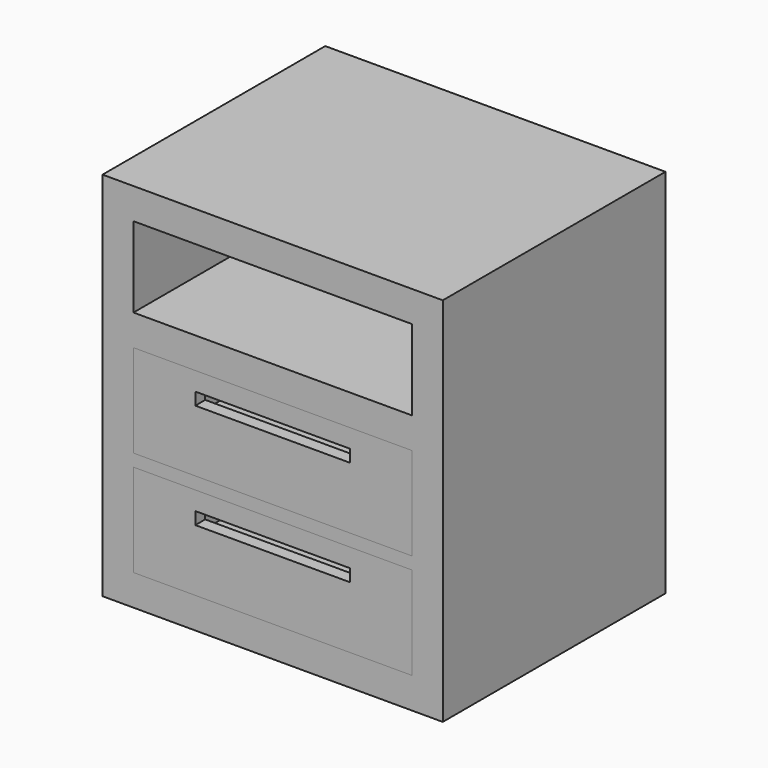
from build123d import *

# Parameters (mm, degrees)
F0_W     = 550
F0_H     = 450
F1_DEPTH = 600
F2_W     = 450
F2_H     = 150
F2_H_2   = 130
F3_DEPTH = 430
F4_DEPTH = 20.001
F5_DEPTH = 430
F6_T     = -20
F6_2_T   = -20
F7_W     = 250
F7_H     = 20
F8_DEPTH = 20


with BuildPart() as f1:
    # F0 (on Top) → F1 (new body)
    with BuildSketch(Plane.XY):
        Rectangle(F0_W, F0_H)
    extrude(amount=F1_DEPTH)

    # F2 (on face) → F3 (cut)
    with BuildSketch(Plane.XZ.offset(225)):
        with Locations((0, 125)):
            Rectangle(F2_W, F2_H)
        with Locations((0, 295)):
            Rectangle(F2_W, F2_H)
        with Locations((0, 485)):
            Rectangle(F2_W, F2_H_2)
    extrude(amount=-F3_DEPTH, mode=Mode.SUBTRACT)

    # F4 (cut, through all): a face of the model
    f4_faces = [f1.faces().sort_by_distance(p)[0] for p in [
        (0, 205, 485),
    ]]
    extrude(f4_faces, amount=-F4_DEPTH, mode=Mode.SUBTRACT)


with BuildPart() as f5:
    # F2 (on face) → F5 (new body, through all)
    with BuildSketch(Plane.XZ.offset(225)):
        with Locations((0, 125)):
            Rectangle(F2_W, F2_H)
    extrude(amount=-F5_DEPTH)

    # F6#2
    f6_2_openings = [f5.faces().sort_by_distance(p)[0] for p in [
        (0, -10, 200),
    ]]
    offset(amount=F6_2_T, openings=f6_2_openings)


with BuildPart() as f5b:
    # F2 (on face) → F5, piece 2 (new body, through all)
    with BuildSketch(Plane.XZ.offset(225)):
        with Locations((0, 295)):
            Rectangle(F2_W, F2_H)
    extrude(amount=-F5_DEPTH)

    # F6
    f6_openings = [f5b.faces().sort_by_distance(p)[0] for p in [
        (0, -10, 370),
    ]]
    offset(amount=F6_T, openings=f6_openings)


with BuildPart() as f8_tool:
    # F7 (on face) → F8 (new body, through all)
    with BuildSketch(Plane.XZ.offset(225)):
        with Locations((0, 330)):
            Rectangle(F7_W, F7_H)
        with Locations((0, 160)):
            Rectangle(F7_W, F7_H)
    extrude(amount=-F8_DEPTH)


with BuildPart() as f5_1:
    add(f5.part)

    # F8: cut by f8_tool
    add(f8_tool.part, mode=Mode.SUBTRACT)


with BuildPart() as f5b_1:
    add(f5b.part)

    # F8: cut by f8_tool
    add(f8_tool.part, mode=Mode.SUBTRACT)


solid = Compound([f1.part, f5_1.part, f5b_1.part])
